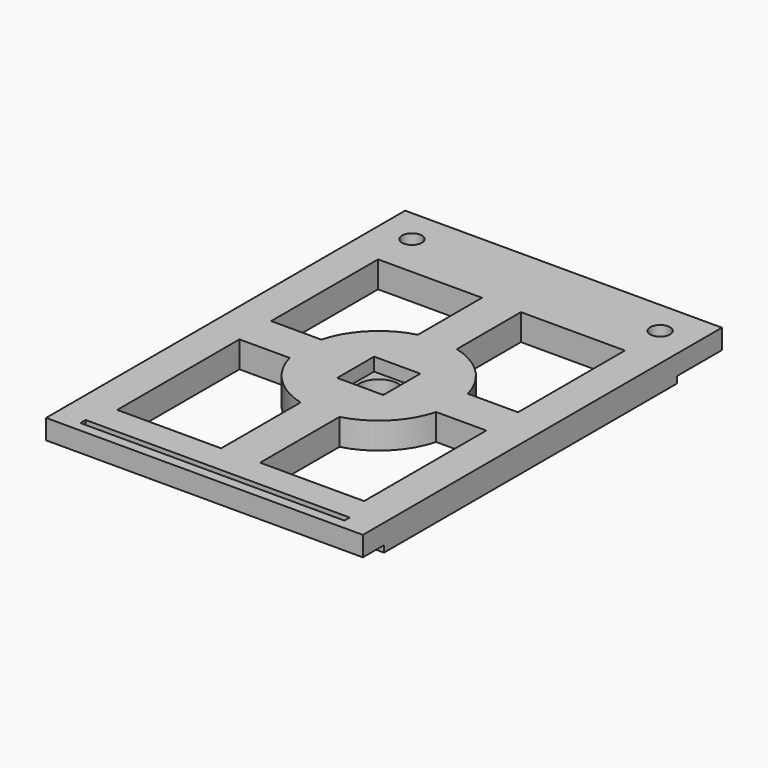
from build123d import *

# Parameters (mm, degrees)
F0_R      = 2.95
F1_DEPTH  = 4
F2_W      = 8.5
F2_H      = 8.5
F3_DEPTH  = 1
F4_R      = 1.5
F5_DEPTH  = 3
F7_DEPTH  = 4
F8_R      = 1.5
F9_DEPTH  = 3
F10_W     = 48
F10_H     = 4
F11_DEPTH = 1
F12_W     = 40
F12_H     = 1
F13_DEPTH = 3
F14_W     = 7
F14_H     = 7
F14_R     = 2.95
F15_DEPTH = 2


# Not quite as in the source:
# - a feature names something its author has since deleted; it is built from what else it names


with BuildPart() as f1:
    # F0 (on Top) → F1 (new body)
    with BuildSketch(Plane.XY):
        Polygon((-24, -33), (24, -33), (24, 26.5), (24, 35), (17.5, 35), (-17.5, 35), (-24, 35), (-24, 26.5), align=None)
        Circle(F0_R, mode=Mode.SUBTRACT)
    extrude(amount=F1_DEPTH)

    # F2 (on face) → F3 (cut)
    with BuildSketch(Plane(origin=(0, 0, 0), x_dir=(1, 0, 0), z_dir=(0, 0, -1))):
        with Locations((19.75, -30.75)):
            Rectangle(F2_W, F2_H)
        with Locations((-19.75, -30.75)):
            Rectangle(F2_W, F2_H)
    extrude(amount=-F3_DEPTH, mode=Mode.SUBTRACT)

    # F4 (on face) → F5 (cut)
    with BuildSketch(Plane(origin=(0, 0, 1), x_dir=(1, 0, 0), z_dir=(0, 0, -1))):
        with Locations((18.7980970389, -29.7980970389)):
            Circle(F4_R)
    extrude(amount=-F5_DEPTH, mode=Mode.SUBTRACT)

    # F6 (on face) → F7 (cut)
    with BuildSketch(Plane.XY.offset(4)):
        with BuildLine():
            Line((-18.7027541446, 3), (-11.1018016556, 3))
            ThreePointArc((-11.1018016556, 3), (-8.1134067433, 8.1500080379), (-2.95, 11.115192306))
            Line((-2.95, 11.115192306), (-2.95, 23.25))
            Line((-2.95, 23.25), (-18.7027541446, 23.25))
            Line((-18.7027541446, 23.25), (-18.7027541446, 3))
        make_face()
        with BuildLine():
            Line((2.95, 23.25), (2.95, 11.115192306))
            ThreePointArc((2.95, 11.115192306), (8.1134067433, 8.1500080379), (11.1018016556, 3))
            Line((11.1018016556, 3), (18.7027541446, 3))
            Line((18.7027541446, 3), (18.7027541446, 23.25))
            Line((18.7027541446, 23.25), (2.95, 23.25))
        make_face()
        with BuildLine():
            Line((-18.7027541446, -9.125), (-18.7027541446, -16.125))
            Line((-18.7027541446, -16.125), (-18.7027541446, -26.1487078986))
            Line((-18.7027541446, -26.1487078986), (-10, -26.1487078986))
            Line((-10, -26.1487078986), (-2.95, -26.1487078986))
            Line((-2.95, -26.1487078986), (-2.95, -11.115192306))
            ThreePointArc((-2.95, -11.115192306), (-8.1134067433, -8.1500080379), (-11.1018016556, -3))
            Line((-11.1018016556, -3), (-17.7254807204, -3))
            Line((-17.7254807204, -3), (-18.7027541446, -3))
            Line((-18.7027541446, -3), (-18.7027541446, -9.125))
        make_face()
        with BuildLine():
            ThreePointArc((11.1018016556, -3), (8.1134067433, -8.1500080379), (2.95, -11.115192306))
            Line((2.95, -11.115192306), (2.95, -26.1487078986))
            Line((2.95, -26.1487078986), (10, -26.1487078986))
            Line((10, -26.1487078986), (18.7027541446, -26.1487078986))
            Line((18.7027541446, -26.1487078986), (18.7027541446, -16.125))
            Line((18.7027541446, -16.125), (18.7027541446, -9.125))
            Line((18.7027541446, -9.125), (18.7027541446, -3.9093415253))
            Line((18.7027541446, -3.9093415253), (18.7027541446, -3))
            Line((18.7027541446, -3), (11.1018016556, -3))
        make_face()
    extrude(amount=-F7_DEPTH, mode=Mode.SUBTRACT)

    # F8 (on face) → F9 (cut)
    with BuildSketch(Plane(origin=(0, 0, 1), x_dir=(1, 0, 0), z_dir=(0, 0, -1))):
        with Locations((-18.7980970389, -29.7980970389)):
            Circle(F8_R)
    extrude(amount=-F9_DEPTH, mode=Mode.SUBTRACT)

    # F10 (on face) → F11 (cut)
    with BuildSketch(Plane(origin=(0, 0, 0), x_dir=(1, 0, 0), z_dir=(0, 0, -1))):
        with Locations((0, 31)):
            Rectangle(F10_W, F10_H)
    extrude(amount=-F11_DEPTH, mode=Mode.SUBTRACT)

    # F12 (on face) → F13 (cut)
    with BuildSketch(Plane(origin=(0, 0, 1), x_dir=(1, 0, 0), z_dir=(0, 0, -1))):
        with Locations((0, 31)):
            Rectangle(F12_W, F12_H)
    extrude(amount=-F13_DEPTH, mode=Mode.SUBTRACT)

    # F14 (on face) → F15 (cut)
    with BuildSketch(Plane.XY.offset(4)):
        Rectangle(F14_W, F14_H)
        Circle(F14_R, mode=Mode.SUBTRACT)
    extrude(amount=-F15_DEPTH, mode=Mode.SUBTRACT)


solid = f1.part
